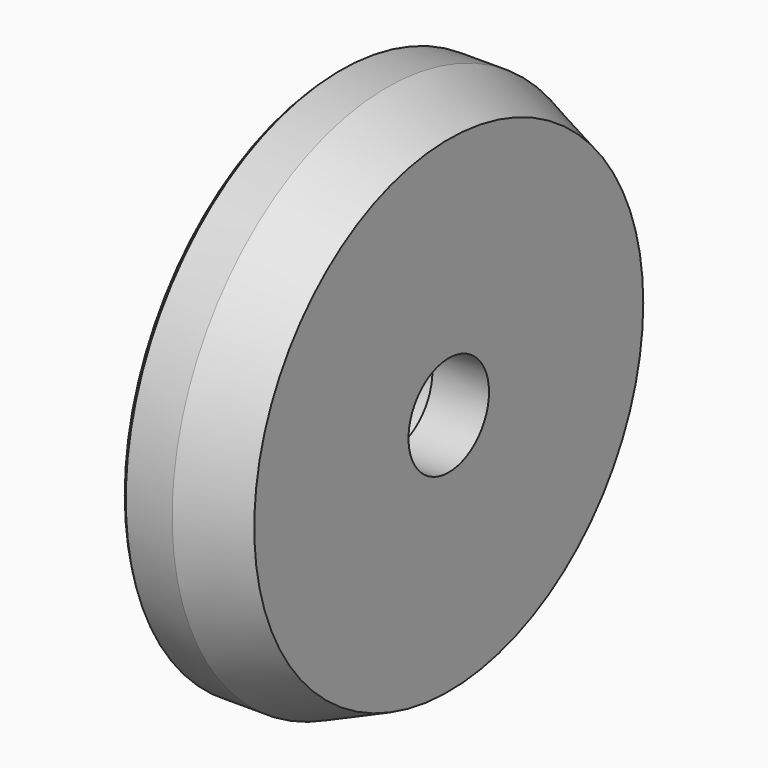
from build123d import *

# Parameters (mm, degrees)
F0_R           = 60.325
F1_DEPTH       = 25.4
F2_SIZE        = 1.143
F4_D           = 22.606
F4_CBORE_D     = 38.1
F4_CBORE_DEPTH = 12.7


# Not quite as in the source:
# - a fillet or chamfer that OpenCascade refuses, or shapes differently, is made with other operations: its cross-section is extruded or revolved along the edge and cut away or added


with BuildPart() as f1:
    # F0 (on Right) → F1 (new body)
    with BuildSketch(Plane.YZ):
        Circle(F0_R)
    extrude(amount=-F1_DEPTH)

    # F2
    f2_edges = [f1.edges().sort_by_distance(p)[0] for p in [
        (-25.4, -60.325, 0),
        (-12.7, 60.325, 0),
        (0, -60.325, 0),
    ]]
    chamfer(f2_edges, length=F2_SIZE)

    # F4 (through all)
    with Locations(Plane(origin=(-25.4, 0, 0), x_dir=(0, -1, 0), z_dir=(-1, 0, 0))):
        with Locations((0, 0)):
            CounterBoreHole(F4_D / 2, F4_CBORE_D / 2, F4_CBORE_DEPTH)

    # F5: chamfer of 12.7 on 1 edges, made by hand

    # F5_s1 → F5_t2 (revolve, cut)
    with BuildSketch(Plane.XY):
        Polygon((-13.843, 60.325), (7.8372561211, 51.3447438789), (-1.143, 60.325), align=None)
    revolve(axis=Axis((-1.143, 0, 0), (1, 0, 0)), mode=Mode.SUBTRACT)


solid = f1.part
